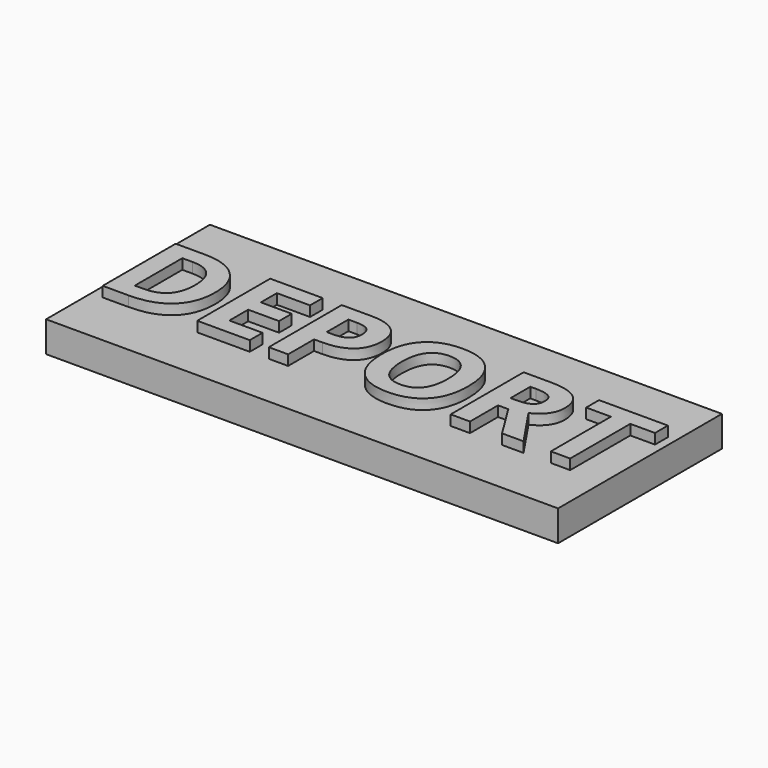
from build123d import *

# Parameters (mm, degrees)
F0_W         = 50
F0_H         = 20
F1_DEPTH     = 3
F2_TEXT_SIZE = 12.4741745605
F3_DEPTH     = 1


# Not quite as in the source:
# - Text() gives the source's letters only with a copy of the font that has no kerning and outlines rounded to 1/6400 em; it was checked with that copy


with BuildPart() as f1:
    # F0 (on Top) → F1 (new body)
    with BuildSketch(Plane.XY):
        Rectangle(F0_W, F0_H)
    extrude(amount=-F1_DEPTH)

    # F2 (on Top) → F3 (join)
    with BuildSketch(Plane.XY):
        with Locations((-25, -4.4907028418)):
            Text('DEPORT', F2_TEXT_SIZE, font='Open Sans', font_style=FontStyle.BOLD, text_align=(TextAlign.LEFT, TextAlign.BOTTOM))
    extrude(amount=F3_DEPTH)


solid = f1.part
